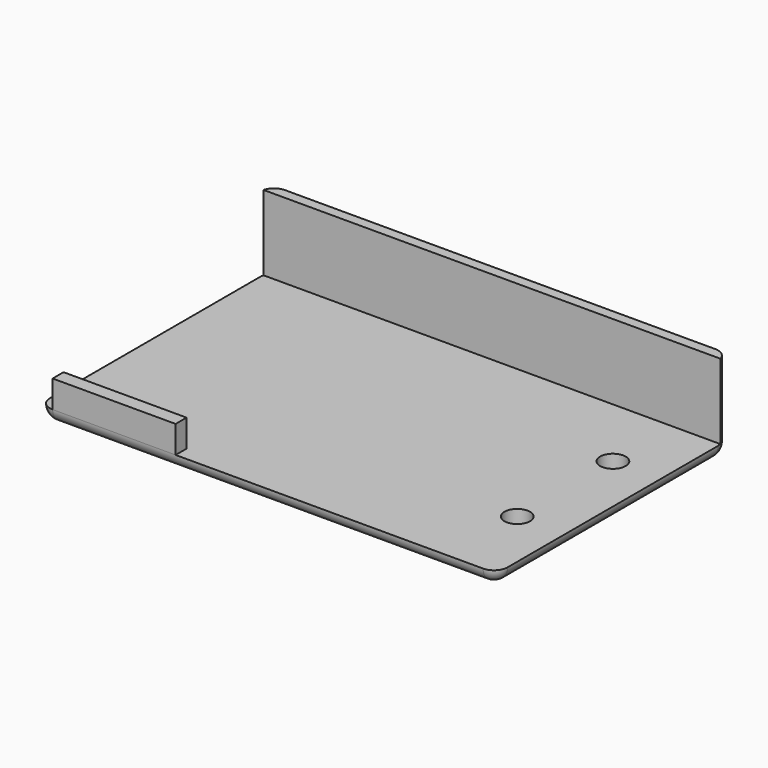
from build123d import *

# Parameters (mm, degrees)
F0_W     = 134
F0_H     = 3
F0_W_2   = 36
F0_H_2   = 4
F0_R     = 3.75
F1_DEPTH = 4
F2_DEPTH = 26
F3_DEPTH = 12
F4_R     = 3.99999


# Not quite as in the source:
# - a fillet or chamfer is up to 0.001 mm smaller than in the source, because OpenCascade refuses the exact size


with BuildPart() as f1:
    # F0 (on Top) → F1 (new body)
    with BuildSketch(Plane.XY):
        with Locations((67, -1.5)):
            Rectangle(F0_W, F0_H)
        with Locations((22, -83)):
            Rectangle(F0_W_2, F0_H_2)
        Polygon((134, -3), (0, -3), (0, -85), (4, -85), (4, -81), (40, -81), (40, -85), (134, -85), align=None)
        with Locations((120, -60)):
            Circle(F0_R, mode=Mode.SUBTRACT)
        with Locations((120, -25)):
            Circle(F0_R, mode=Mode.SUBTRACT)
    extrude(amount=F1_DEPTH)

    # F0 (on Top) → F2 (join)
    with BuildSketch(Plane.XY):
        with Locations((67, -1.5)):
            Rectangle(F0_W, F0_H)
    extrude(amount=F2_DEPTH)

    # F0 (on Top) → F3 (join)
    with BuildSketch(Plane.XY):
        with Locations((22, -83)):
            Rectangle(F0_W_2, F0_H_2)
    extrude(amount=F3_DEPTH)

    # F4 (radius 4 in the source; OpenCascade refuses exactly that, so slightly less here)
    f4_edges = [f1.edges().sort_by_distance(p)[0] for p in [
        (67, -85, 0),
        (134, -42.5, 0),
        (0, -42.5, 0),
        (67, 0, 0),
        (134, 0, 13),
        (0, 0, 13),
        (134, -85, 2),
        (0, -85, 2),
    ]]
    fillet(f4_edges, radius=F4_R)


solid = f1.part
